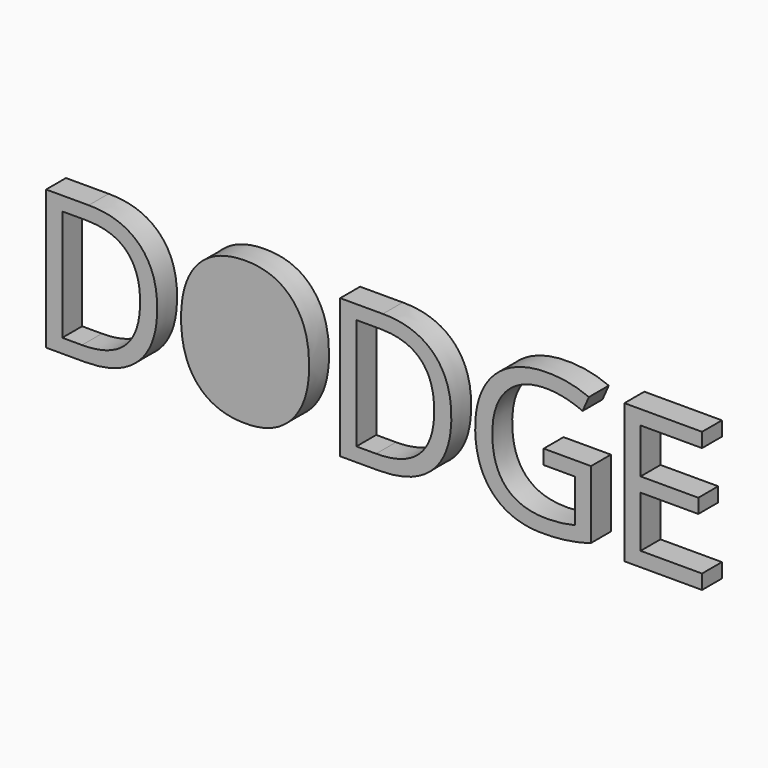
from build123d import *

# Parameters (mm, degrees)
F0_TEXT_SIZE = 49.837720063
F1_DEPTH     = 6.35


# Not quite as in the source:
# - Text() gives the source's letters only with a copy of the font that has no kerning and outlines rounded to 1/6400 em; it was checked with that copy


with BuildPart() as f1:
    # F0 (on Front) → F1 (new body)
    with BuildSketch(Plane.XZ):
        with BuildLine():
            add(Edge.make_bspline(
                [(10.9526176982, 11.470056928), (7.8728023412, 7.7322279232), (7.8728023412, 0.606991383)],
                knots=[0, 0, 0, 1, 1, 1], degree=2))
            add(Edge.make_bspline(
                [(7.8728023412, 0.606991383), (7.8728023412, -6.6194780261), (10.9526176982, -10.3573070309)],
                knots=[0, 0, 0, 1, 1, 1], degree=2))
            add(Edge.make_bspline(
                [(10.9526176982, -10.3573070309), (14.0324330552, -14.0951360356), (19.8961523064, -14.0951360356)],
                knots=[0, 0, 0, 1, 1, 1], degree=2))
            add(Edge.make_bspline(
                [(19.8961523064, -14.0951360356), (25.8065944201, -14.0951360356), (28.8241126271, -10.3728813184)],
                knots=[0, 0, 0, 1, 1, 1], degree=2))
            add(Edge.make_bspline(
                [(28.8241126271, -10.3728813184), (31.841630834, -6.6506266012), (31.841630834, 0.606991383)],
                knots=[0, 0, 0, 1, 1, 1], degree=2))
            add(Edge.make_bspline(
                [(31.841630834, 0.606991383), (31.841630834, 7.7867379296), (28.8357933427, 11.4973119311)],
                knots=[0, 0, 0, 1, 1, 1], degree=2))
            add(Edge.make_bspline(
                [(28.8357933427, 11.4973119311), (25.8299558514, 15.2078859327), (19.942875169, 15.2078859327)],
                knots=[0, 0, 0, 1, 1, 1], degree=2))
            add(Edge.make_bspline(
                [(19.942875169, 15.2078859327), (14.0324330552, 15.2078859327), (10.9526176982, 11.470056928)],
                knots=[0, 0, 0, 1, 1, 1], degree=2))
        make_face()
        with Locations((-35.8831584454, -17.2333549708)):
            Text('DODGE', F0_TEXT_SIZE, font='Open Sans', text_align=(TextAlign.LEFT, TextAlign.BOTTOM))
    extrude(amount=F1_DEPTH)


solid = f1.part
